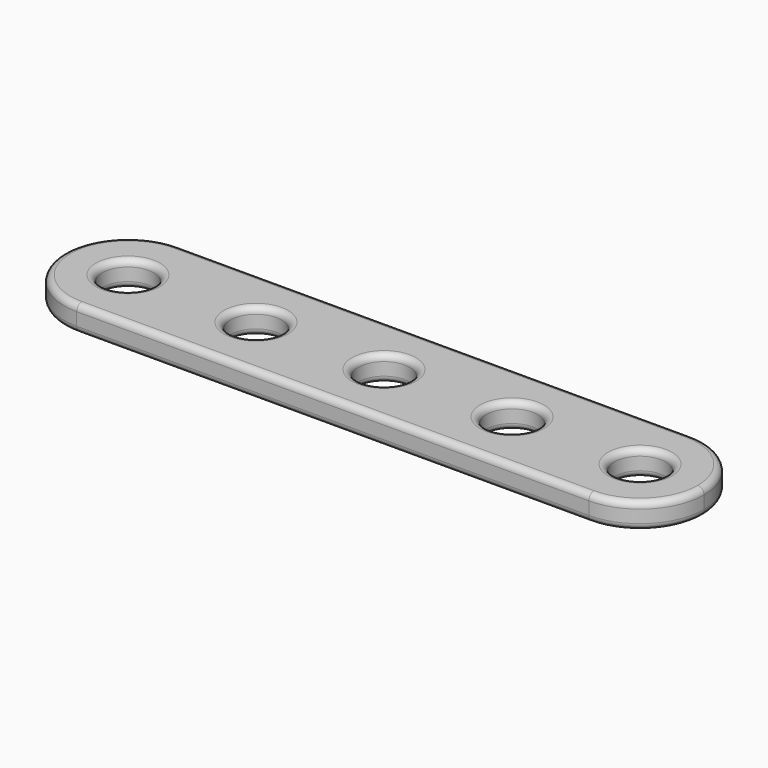
from build123d import *

# Parameters (mm, degrees)
F0_W     = 50
F0_H     = 10
F1_DEPTH = 2
F3_R     = 2
F2_DEPTH = 25
F4_R     = 4.99999
F5_R     = 2
F6_DEPTH = 25
F7_R     = 0.5


# Not quite as in the source:
# - a fillet or chamfer is up to 0.001 mm smaller than in the source, because OpenCascade refuses the exact size


with BuildPart() as f1:
    # F0 (on Top) → F1 (new body)
    with BuildSketch(Plane.XY):
        Rectangle(F0_W, F0_H)
    extrude(amount=F1_DEPTH)

    # F3 (on Top) → F2 (cut)
    with BuildSketch(Plane.XY):
        with Locations((-20, 0)):
            Circle(F3_R)
        with Locations((-10, 0)):
            Circle(F3_R)
        Circle(F3_R)
        with Locations((10, 0)):
            Circle(F3_R)
        with Locations((20, 0)):
            Circle(F3_R)
    extrude(amount=-F2_DEPTH, mode=Mode.SUBTRACT)

    # F4 (radius 5 in the source; OpenCascade refuses exactly that, so slightly less here)
    f4_edges = [f1.edges().sort_by_distance(p)[0] for p in [
        (25, -5, 1),
        (25, 5, 1),
        (-25, -5, 1),
        (-25, 5, 1),
    ]]
    fillet(f4_edges, radius=F4_R)

    # F5 (on face) → F6 (cut)
    with BuildSketch(Plane.XY.offset(2)):
        with Locations((20, 0)):
            Circle(F5_R)
        with Locations((10, 0)):
            Circle(F5_R)
        Circle(F5_R)
        with Locations((-10, 0)):
            Circle(F5_R)
        with Locations((-20, 0)):
            Circle(F5_R)
    extrude(amount=-F6_DEPTH, mode=Mode.SUBTRACT)

    # F7
    f7_edges = [f1.edges().sort_by_distance(p)[0] for p in [
        (25, 0, 2),
        (23.535537, -3.535537, 2),
        (23.535537, 3.535537, 2),
        (0, -5, 2),
        (0, 5, 2),
        (-23.535537, -3.535537, 2),
        (-23.535537, 3.535537, 2),
        (-25, 0, 2),
        (-22, 0, 2),
        (-12, 0, 2),
        (-2, 0, 2),
        (8, 0, 2),
        (18, 0, 2),
        (25, 0, 0),
        (23.535537, -3.535537, 0),
        (23.535537, 3.535537, 0),
        (0, -5, 0),
        (0, 5, 0),
        (-23.535537, -3.535537, 0),
        (-23.535537, 3.535537, 0),
        (-25, 0, 0),
        (-22, 0, 0),
        (-12, 0, 0),
        (-2, 0, 0),
        (8, 0, 0),
        (18, 0, 0),
    ]]
    fillet(f7_edges, radius=F7_R)


solid = f1.part
